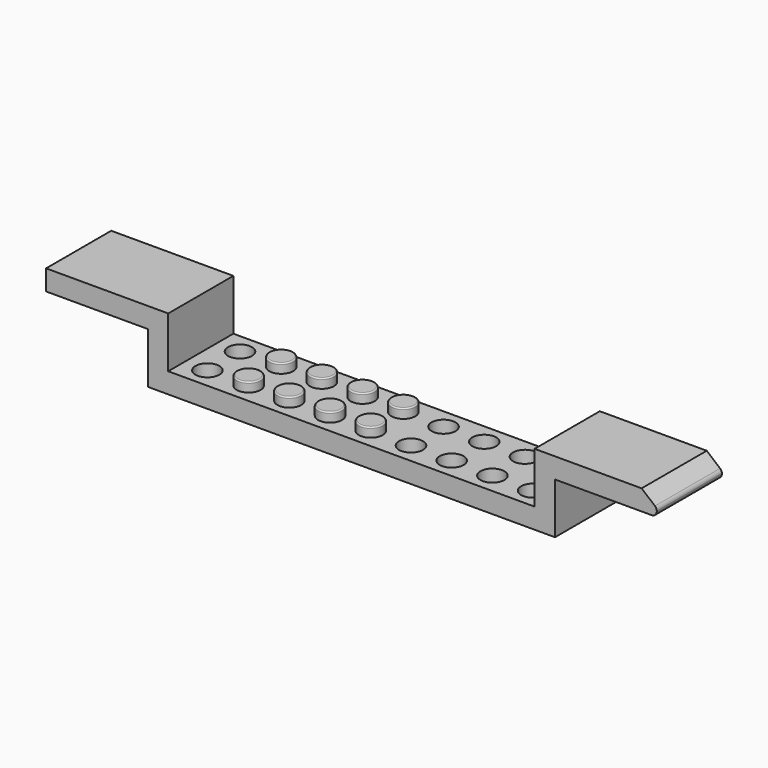
from build123d import *

# Parameters (mm, degrees)
F1_DEPTH  = 16
F2_W      = 13.0048
F2_H      = 13
F2_R      = 3.3
F2_R_2    = 2.4003
F3_DEPTH  = 3
F5_R      = 2.35
F6_DEPTH  = 1.85
F7_SIZE2  = 2.5
F7_SIZE   = 2.9793839815
F8_R      = 0.25
F9_SIZE   = 0.2
F10_R     = 1
F11_R     = 2.35
F12_DEPTH = 25


# Not quite as in the source:
# - a feature names something its author has since deleted; it is built from what else it names


with BuildPart() as f1:
    # F0 (on Front) → F1 (new body)
    with BuildSketch(Plane.XZ):
        Polygon((-40, 0), (0, 0), (0, 4), (-36, 4), (-36, 14), (-60, 14), (-60, 10), (-40, 10), align=None)
    extrude(amount=-F1_DEPTH)

    # F2 (on face) → F3 (cut)
    with BuildSketch(Plane(origin=(0, 0, 10), x_dir=(1, 0, 0), z_dir=(0, 0, -1))):
        with Locations((-50, -8)):
            Rectangle(F2_W, F2_H)
        with Locations((-50, -8)):
            Circle(F2_R, mode=Mode.SUBTRACT)
        with Locations((-50, -8)):
            Circle(F2_R_2)
    extrude(amount=-F3_DEPTH, mode=Mode.SUBTRACT)

    # F4: F1 across face


with BuildPart() as f1_1:
    add(f1.part)
    add(f1.part.mirror(Plane(origin=(0, 8, 2), x_dir=(0, 1, 0), z_dir=(1, 0, 0))))

    # F5 (on face) → F6 (join)
    with BuildSketch(Plane.XY.offset(4)):
        with Locations((-23.3999874801, 4)):
            Circle(F5_R)
        with Locations((-23.3999874801, 12)):
            Circle(F5_R)
        with Locations((-15.3999874801, 12)):
            Circle(F5_R)
        with Locations((-15.3999874801, 4)):
            Circle(F5_R)
        with Locations((-7.3999874801, 4)):
            Circle(F5_R)
        with Locations((-7.3999874801, 12)):
            Circle(F5_R)
        with Locations((0.6000125199, 12)):
            Circle(F5_R)
        with Locations((0.6000125199, 4)):
            Circle(F5_R)
    extrude(amount=F6_DEPTH)

    # F7
    f7_edges = [f1_1.edges().sort_by_distance(p)[0] for p in [
        (60, 8, 14),
    ]]
    f7_side = f1_1.faces().sort_by_distance((48, 8, 14))[0]
    chamfer(f7_edges, length=F7_SIZE, length2=F7_SIZE2, reference=f7_side)

    # F8
    f8_edges = [f1_1.edges().sort_by_distance(p)[0] for p in [
        (-25.749987, 4, 5.85),
        (-25.749987, 12, 5.85),
        (-17.749987, 12, 5.85),
        (-17.749987, 4, 5.85),
        (-9.749987, 4, 5.85),
        (-9.749987, 12, 5.85),
        (-1.749987, 12, 5.85),
        (-1.749987, 4, 5.85),
    ]]
    fillet(f8_edges, radius=F8_R)

    # F9
    f9_edges = [f1_1.edges().sort_by_distance(p)[0] for p in [
        (-53.3, 8, 10),
    ]]
    chamfer(f9_edges, length=F9_SIZE)

    # F10
    f10_edges = [f1_1.edges().sort_by_distance(p)[0] for p in [
        (60, 8, 11.5),
        (60, 8, 10),
    ]]
    fillet(f10_edges, radius=F10_R)

    # F11 (on face) → F12 (cut)
    with BuildSketch(Plane.XY.offset(4)):
        with Locations((-31.4999707043, 4)):
            Circle(F11_R)
        with Locations((-31.4999707043, 12)):
            Circle(F11_R)
        with Locations((8.5000292957, 12)):
            Circle(F11_R)
        with Locations((8.5000292957, 4)):
            Circle(F11_R)
        with Locations((16.5000292957, 4)):
            Circle(F11_R)
        with Locations((16.5000292957, 12)):
            Circle(F11_R)
        with Locations((24.5000292957, 12)):
            Circle(F11_R)
        with Locations((24.5000292957, 4)):
            Circle(F11_R)
        with Locations((32.5000292957, 4)):
            Circle(F11_R)
        with Locations((32.5000292957, 12)):
            Circle(F11_R)
    extrude(amount=-F12_DEPTH, mode=Mode.SUBTRACT)


solid = f1_1.part
